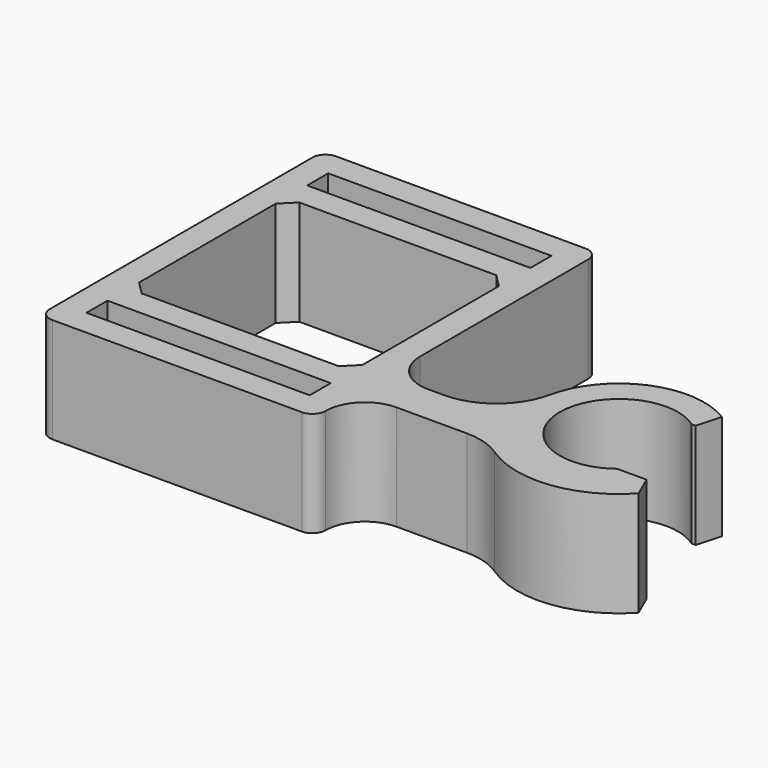
from build123d import *

# Parameters (mm, degrees)
F0_W        = 17
F0_H        = 2
F0_H_2      = 15
F1_DEPTH    = 8
F2_R        = 5
F3_T1_DEPTH = 8
F3_T3_DEPTH = 18.3525106995
F3_T5_DEPTH = 21.4805273161
F4_R        = 1
F5_R        = 2.99999


# Not quite as in the source:
# - a fillet or chamfer that OpenCascade refuses, or shapes differently, is made with other operations: its cross-section is extruded or revolved along the edge and cut away or added
# - a fillet or chamfer is up to 0.001 mm smaller than in the source, because OpenCascade refuses the exact size


with BuildPart() as f1:
    # F0 (on Top) → F1 (new body)
    with BuildSketch(Plane.XY):
        with BuildLine():
            ThreePointArc((2.7332443879, -3.5748251868), (-4.4992296638, -0.0832612306), (2.5991092476, 3.6735039294))
            Line((2.5991092476, 3.6735039294), (5.3624032747, 3.6735039294))
            ThreePointArc((5.3624032747, 3.6735039294), (-3.1508257353, 5.6852701946), (-5.9573484034, -2.6))
            Line((-5.9573484034, -2.6), (-15.4573484034, -2.6))
            Line((-15.4573484034, -2.6), (-15.4573484034, 13.4))
            Line((-15.4573484034, 13.4), (-15.4573484034, 17.4032363431))
            Line((-15.4573484034, 17.4032363431), (-36.4629774356, 17.4032363431))
            Line((-36.4629774356, 17.4032363431), (-36.4629774356, 11.4032363431))
            Line((-36.4629774356, 11.4032363431), (-36.4629774356, -9.5967636569))
            Line((-36.4629774356, -9.5967636569), (-15.4629774356, -9.5967636569))
            Line((-15.4629774356, -9.5967636569), (-15.4629774356, -5.5967636569))
            Line((-15.4629774356, -5.5967636569), (-5.3631004506, -5.5967636569))
            ThreePointArc((-5.3631004506, -5.5967636569), (1.2632530504, -7.6479279289), (6.8780254985, -3.5748251868))
            Line((6.8780254985, -3.5748251868), (2.7332443879, -3.5748251868))
        make_face()
        with Locations((-25.9629774356, -6.6)):
            Rectangle(F0_W, F0_H, mode=Mode.SUBTRACT)
        with Locations((-25.9573484034, 3.9)):
            Rectangle(F0_W, F0_H_2, mode=Mode.SUBTRACT)
        with Locations((-25.9573484034, 14.4032363431)):
            Rectangle(F0_W, F0_H, mode=Mode.SUBTRACT)
    extrude(amount=F1_DEPTH)

    # F2
    f2_edges = [f1.edges().sort_by_distance(p)[0] for p in [
        (-5.957348, -2.6, 4),
        (-5.3631, -5.596764, 4),
    ]]
    fillet(f2_edges, radius=F2_R)

    # F3: chamfer of 1 on 6 edges, made by hand

    # F3_s2 → F3_t1 (join)
    with BuildSketch(Plane.XY):
        Polygon((-34.4573484034, -2.6), (-33.4573484034, -3.6), (-34.4573484034, -3.6), align=None)
        Polygon((-34.4573484034, 10.4), (-33.4573484034, 11.4), (-34.4573484034, 11.4), align=None)
        Polygon((-18.4573484034, 11.4), (-17.4573484034, 10.4), (-17.4573484034, 11.4), align=None)
        Polygon((-17.4573484034, -2.6), (-18.4573484034, -3.6), (-17.4573484034, -3.6), align=None)
    extrude(amount=F3_T1_DEPTH)

    # F3_s4 → F3_t3 (cut)
    with BuildSketch(Plane.XY.offset(-5.1762553498)):
        with BuildLine():
            Line((5.7007617196, -5.2524209363), (4.9653271539, -3.5748251868))
            Line((4.9653271539, -3.5748251868), (6.8780254985, -3.5748251868))
            ThreePointArc((6.8780254985, -3.5748251868), (6.3390727508, -4.4612516781), (5.7007617196, -5.2524209363))
        make_face()
    extrude(amount=F3_T3_DEPTH, mode=Mode.SUBTRACT)

    # F3_s6 → F3_t5 (cut)
    with BuildSketch(Plane.XY.offset(-6.740263658)):
        with BuildLine():
            Line((2.8997174039, 3.6735039294), (3.42693875, 5.5232319165))
            ThreePointArc((3.42693875, 5.5232319165), (4.4840607821, 4.7056560544), (5.3624032747, 3.6735039294))
            Line((5.3624032747, 3.6735039294), (2.8997174039, 3.6735039294))
        make_face()
    extrude(amount=F3_T5_DEPTH, mode=Mode.SUBTRACT)

    # F4
    f4_edges = [f1.edges().sort_by_distance(p)[0] for p in [
        (-15.462977, -9.596764, 4),
        (-36.462977, 17.403236, 4),
        (-15.457348, 17.403236, 4),
        (-36.462977, -9.596764, 4),
    ]]
    fillet(f4_edges, radius=F4_R)

    # F5 (radius 3 in the source; OpenCascade refuses exactly that, so slightly less here)
    f5_edges = [f1.edges().sort_by_distance(p)[0] for p in [
        (-15.457348, -2.6, 4),
        (-15.462977, -5.596764, 4),
    ]]
    fillet(f5_edges, radius=F5_R)


solid = f1.part
